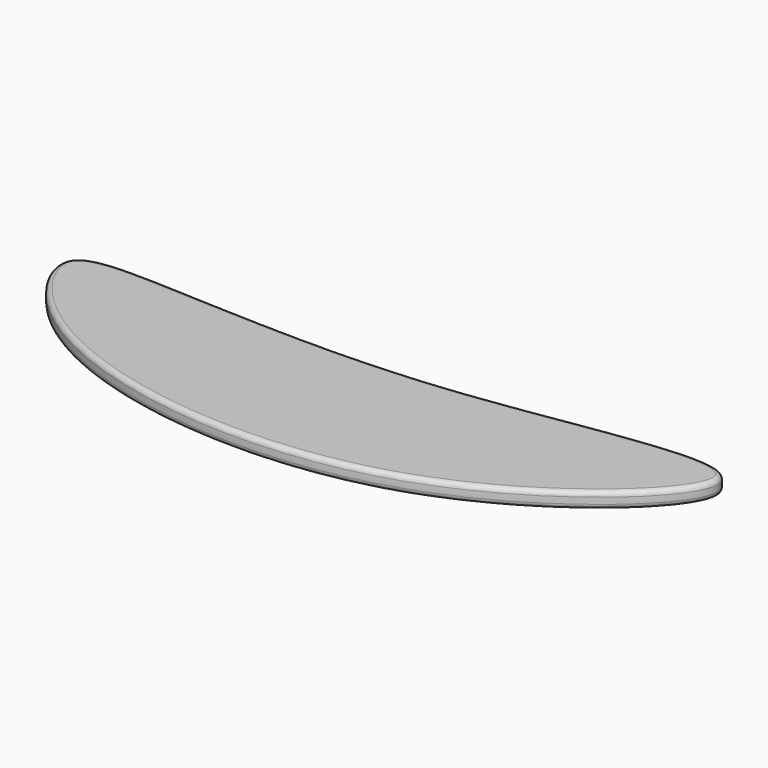
from build123d import *

# Parameters (mm, degrees)
F1_DEPTH = 2.032
F2_R     = 0.6132102448


with BuildPart() as f1:
    # F0 (on Top) → F1 (new body)
    with BuildSketch(Plane.XY):
        with BuildLine():
            add(Edge.make_bspline(
                [(-78.1772732735, -23.5584992915), (-83.0241566888, -23.4194125306), (-91.5394859911, -23.5884961898), (-79.5475976034, -42.9565757843), (-31.2227519064, -49.0504742802), (6.0310408074, -13.7511706378), (-42.7267262231, -25.9940518064), (-68.5370080223, -23.8351375256), (-78.1772732735, -23.5584992915)],
                knots=[0, 0, 0, 0, 0.1000811848, 0.2203853962, 0.4454306317, 0.6198990826, 0.8009423612, 1, 1, 1, 1], degree=3))
        make_face()
    extrude(amount=F1_DEPTH)

    # F2
    f2_edges = [f1.edges().sort_by_distance(p)[0] for p in [
        (-18.50885, -34.395706, 2.032),
        (-18.50885, -34.395706, 0),
    ]]
    fillet(f2_edges, radius=F2_R)


solid = f1.part
